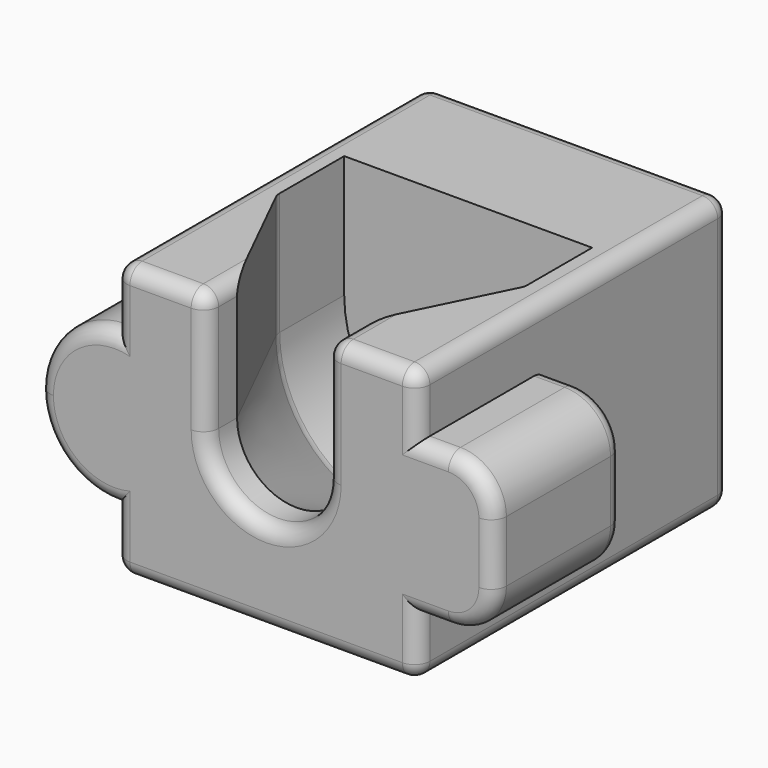
from build123d import *

# Parameters (mm, degrees)
F1_ANGLE = 180
F3_DEPTH = 18.5
F4_DEPTH = 8
F6_DEPTH = 18.5
F7_DEPTH = 8
F5_W     = 5
F5_H     = 10
F8_DEPTH = 7
F9_R     = 1


with BuildPart() as f1:
    # F0 (on Top) → F1 (revolve)
    with BuildSketch(Plane.XY):
        Polygon((-9.9, 18.5), (-9.9, 0), (-3.9, 0), (-3.9, 2.5), (-8.1, 11), (-8.1, 16.5), (0, 16.5), (0, 18.5), align=None)
    revolve(axis=Axis((0, -5.2679181099, 0), (0, -1, 0)), revolution_arc=F1_ANGLE)

    # F2 (on face) → F3 (join, through all)
    with BuildSketch(Plane(origin=(0, 18.5, 0), x_dir=(-1, 0, 0), z_dir=(0, 1, 0))):
        with BuildLine():
            ThreePointArc((4.3e-08, -9.9), (-7.0003571186, -7.0003571489), (-9.9, 0))
            Line((-9.9, 0), (-9.9, -9.9))
            Line((-9.9, -9.9), (4.3e-08, -9.9))
        make_face()
        with BuildLine():
            ThreePointArc((9.9, 0), (7.0003571489, -7.0003571186), (4.3e-08, -9.9))
            Line((4.3e-08, -9.9), (9.9, -9.9))
            Line((9.9, -9.9), (9.9, 0))
        make_face()
    extrude(amount=-F3_DEPTH)

    # F4 (add): a face of the model
    f4_faces = [f1.faces().sort_by_distance(p)[0] for p in [
        (-9.6290221411, 9.25, 0),
    ]]
    extrude(f4_faces, amount=F4_DEPTH)

    # F5 (on face) → F6 (join, through all)
    with BuildSketch(Plane(origin=(0, 18.5, 0), x_dir=(-1, 0, 0), z_dir=(0, 1, 0))):
        with BuildLine():
            ThreePointArc((9.9, -5.95), (13.4355339059, -4.4855339059), (14.9, -0.95))
            ThreePointArc((14.9, -0.95), (13.4355339059, 2.5855339059), (9.9, 4.05))
            Line((9.9, 4.05), (9.9, -5.95))
        make_face()
        with BuildLine():
            Line((-9.9, -5.95), (-9.9, 4.05))
            Line((-9.9, 4.05), (-11.9, 4.05))
            ThreePointArc((-11.9, 4.05), (-14.0213203436, 3.1713203436), (-14.9, 1.05))
            Line((-14.9, 1.05), (-14.9, -2.95))
            ThreePointArc((-14.9, -2.95), (-14.0213203436, -5.0713203436), (-11.9, -5.95))
            Line((-11.9, -5.95), (-9.9, -5.95))
        make_face()
    extrude(amount=-F6_DEPTH)

    # F5 (on face) → F7 (cut)
    with BuildSketch(Plane(origin=(0, 18.5, 0), x_dir=(-1, 0, 0), z_dir=(0, 1, 0))):
        with BuildLine():
            ThreePointArc((9.9, -5.95), (13.4355339059, -4.4855339059), (14.9, -0.95))
            ThreePointArc((14.9, -0.95), (13.4355339059, 2.5855339059), (9.9, 4.05))
            Line((9.9, 4.05), (9.9, -5.95))
        make_face()
        with BuildLine():
            Line((-9.9, -5.95), (-9.9, 4.05))
            Line((-9.9, 4.05), (-11.9, 4.05))
            ThreePointArc((-11.9, 4.05), (-14.0213203436, 3.1713203436), (-14.9, 1.05))
            Line((-14.9, 1.05), (-14.9, -2.95))
            ThreePointArc((-14.9, -2.95), (-14.0213203436, -5.0713203436), (-11.9, -5.95))
            Line((-11.9, -5.95), (-9.9, -5.95))
        make_face()
    extrude(amount=-F7_DEPTH, mode=Mode.SUBTRACT)

    # F5 (on face) → F8 (join)
    with BuildSketch(Plane(origin=(0, 18.5, 0), x_dir=(-1, 0, 0), z_dir=(0, 1, 0))):
        with BuildLine():
            Line((9.9, -5.95), (9.9, 4.05))
            ThreePointArc((9.9, 4.05), (4.9, -0.95), (9.9, -5.95))
        make_face()
        with BuildLine():
            ThreePointArc((9.9, -5.95), (4.9, -0.95), (9.9, 4.05))
            Line((9.9, 4.05), (9.9, 8))
            Line((9.9, 8), (-9.9, 8))
            Line((-9.9, 8), (-9.9, 4.05))
            Line((-9.9, 4.05), (-4.9, 4.05))
            Line((-4.9, 4.05), (-4.9, -5.95))
            Line((-4.9, -5.95), (-9.9, -5.95))
            Line((-9.9, -5.95), (-9.9, -9.9))
            Line((-9.9, -9.9), (9.9, -9.9))
            Line((9.9, -9.9), (9.9, -5.95))
        make_face()
        with Locations((-7.4, -0.95)):
            Rectangle(F5_W, F5_H)
    extrude(amount=F8_DEPTH)

    # F9
    f9_edges = [f1.edges().sort_by_distance(p)[0] for p in [
        (9.9, 12.75, 8),
        (-9.9, 12.75, 8),
        (9.9, 12.75, -9.9),
        (-9.9, 12.75, -9.9),
        (-6.9, 0, 8),
        (9.9, 0, 6.025),
        (9.9, 0, -7.925),
        (-9.9, 0, -7.925),
        (-9.9, 0, 6.025),
        (0, 0, -9.9),
        (0, 0, -3.9),
        (-3.9, 0, 4),
        (-14.9, 0, -0.95),
        (10.9, 0, -5.95),
        (14.02132, 0, -5.07132),
        (14.9, 0, -0.95),
        (14.02132, 0, 3.17132),
        (10.9, 0, 4.05),
        (6.9, 0, 8),
        (3.9, 0, 4),
        (0, 25.5, 8),
        (9.9, 25.5, -0.95),
        (0, 25.5, -9.9),
        (-9.9, 25.5, -0.95),
        (14.9, 10.5, -0.95),
        (-14.9, 10.5, -0.95),
        (-3.9, 1.25, 8),
        (-8.1, 11, 4),
        (3.9, 1.25, 8),
        (10.9, 10.5, -5.95),
        (14.02132, 10.5, -5.07132),
        (14.02132, 10.5, 3.17132),
        (10.9, 10.5, 4.05),
        (0, 11, -8.1),
        (8.1, 11, 4),
    ]]
    fillet(f9_edges, radius=F9_R)


solid = f1.part
